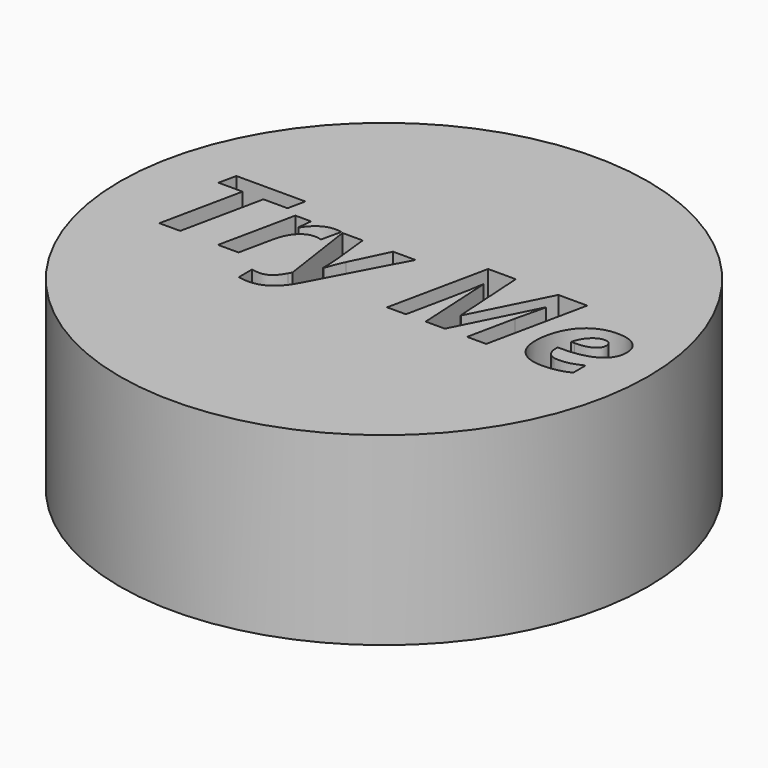
from build123d import *

# Parameters (mm, degrees)
F0_R         = 20
F1_DEPTH     = 14
F2_TEXT_SIZE = 10.6001558846
F3_DEPTH     = 35.306


# Not quite as in the source:
# - Text() gives the source's letters only with a copy of the font that has no kerning and outlines rounded to 1/6400 em; it was checked with that copy


with BuildPart() as f1:
    # F0 (on Top) → F1 (new body)
    with BuildSketch(Plane.XY):
        Circle(F0_R)
    extrude(amount=F1_DEPTH)

    # F2 (on Top) → F3 (cut)
    with BuildSketch(Plane.XY):
        with Locations((-16.2123831874, -2.719400606)):
            Text('Try Me', F2_TEXT_SIZE, font='Open Sans', font_style=FontStyle.BOLDITALIC, text_align=(TextAlign.LEFT, TextAlign.BOTTOM))
    extrude(amount=F3_DEPTH, mode=Mode.SUBTRACT)


solid = f1.part
